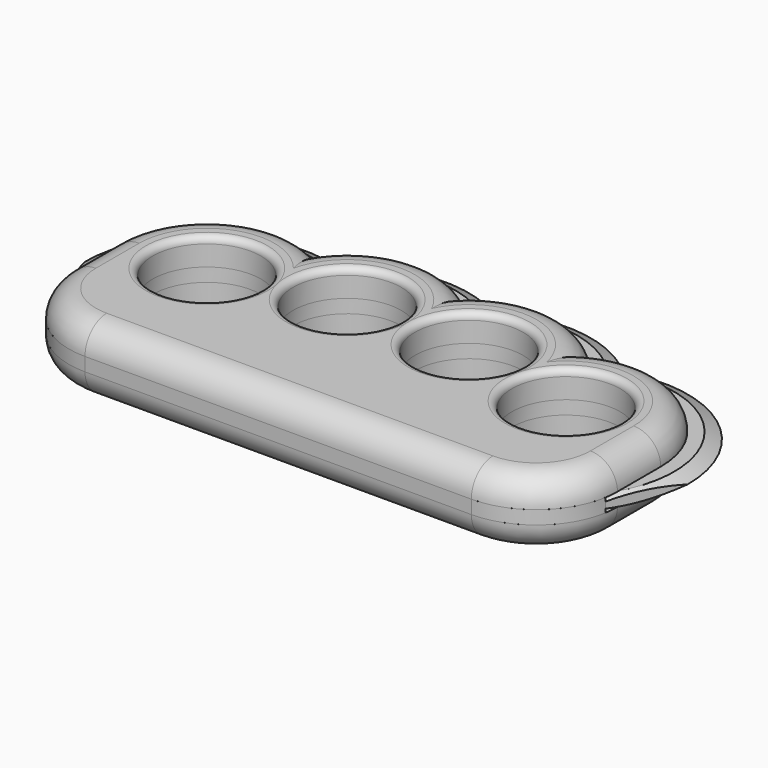
from build123d import *

# Parameters (mm, degrees)
F1_START = 1.5875
F0_R     = 12.7
F1_DEPTH = 6.35
F2_START = -1.5875
F2_DEPTH = 6.35
F3_R     = 12.7
F4_DEPTH = 3.175
F5_SIZE2 = 3.175
F5_SIZE  = 1.5875
F6_SIZE2 = 1.58749
F6_SIZE  = 3.17499
F7_DEPTH = 3.175
F8_R     = 6.34999
F8_2_R   = 6.34999
F9_R     = 1.58749
F9_2_R   = 1.58749


# Not quite as in the source:
# - a fillet or chamfer is up to 0.001 mm smaller than in the source, because OpenCascade refuses the exact size


with BuildPart() as f1:
    # F0 (on Top) → F1 (new body)
    with BuildSketch(Plane.XY.offset(F1_START)):
        with BuildLine():
            ThreePointArc((32.0008761662, 51.5233725194), (16.7725271795, 60.185634809), (0, 55.1240409054))
            ThreePointArc((0, 55.1240409054), (-16.7725271795, 60.185634809), (-32.0008761662, 51.5233725194))
            ThreePointArc((-32.0008761662, 51.5233725194), (-53.7331431906, 50.7166907676), (-64.37301193, 31.75))
            Line((-64.37301193, 31.75), (-64.37301193, 19.05))
            ThreePointArc((-64.37301193, 19.05), (-58.7933961116, 5.5796158184), (-45.32301193, 0))
            Line((-45.32301193, 0), (0, 0))
            Line((0, 0), (45.32301193, 0))
            ThreePointArc((45.32301193, 0), (58.7933961116, 5.5796158184), (64.37301193, 19.05))
            Line((64.37301193, 19.05), (64.37301193, 31.75))
            ThreePointArc((64.37301193, 31.75), (53.7331431906, 50.7166907676), (32.0008761662, 51.5233725194))
        make_face()
        with Locations((-42.14801193, 31.75)):
            Circle(F0_R, mode=Mode.SUBTRACT)
        with Locations((-14.2875, 38.1)):
            Circle(F0_R, mode=Mode.SUBTRACT)
        with Locations((14.2875, 38.1)):
            Circle(F0_R, mode=Mode.SUBTRACT)
        with Locations((42.14801193, 31.75)):
            Circle(F0_R, mode=Mode.SUBTRACT)
    extrude(amount=F1_DEPTH)

    # F8 (radius 6.35 in the source; OpenCascade refuses exactly that, so slightly less here)
    f8_edges = [f1.edges().sort_by_distance(p)[0] for p in [
        (-58.793396, 5.579616, 7.9375),
        (-64.373012, 25.4, 7.9375),
        (-53.733143, 50.716691, 7.9375),
        (-16.772527, 60.185635, 7.9375),
        (16.772527, 60.185635, 7.9375),
        (53.733143, 50.716691, 7.9375),
        (58.793396, 5.579616, 7.9375),
        (64.373012, 25.4, 7.9375),
        (0, 0, 7.9375),
    ]]
    fillet(f8_edges, radius=F8_R)

    # F9#2 (radius 1.5875 in the source; OpenCascade refuses exactly that, so slightly less here)
    f9_2_edges = [f1.edges().sort_by_distance(p)[0] for p in [
        (29.448012, 31.75, 7.9375),
        (1.5875, 38.1, 7.9375),
        (-26.9875, 38.1, 7.9375),
        (-54.848012, 31.75, 7.9375),
    ]]
    fillet(f9_2_edges, radius=F9_2_R)


with BuildPart() as f2:
    # F0 (on Top) → F2 (new body)
    with BuildSketch(Plane.XY.offset(F2_START)):
        with BuildLine():
            ThreePointArc((32.0008761662, 51.5233725194), (16.7725271795, 60.185634809), (0, 55.1240409054))
            ThreePointArc((0, 55.1240409054), (-16.7725271795, 60.185634809), (-32.0008761662, 51.5233725194))
            ThreePointArc((-32.0008761662, 51.5233725194), (-53.7331431906, 50.7166907676), (-64.37301193, 31.75))
            Line((-64.37301193, 31.75), (-64.37301193, 19.05))
            ThreePointArc((-64.37301193, 19.05), (-58.7933961116, 5.5796158184), (-45.32301193, 0))
            Line((-45.32301193, 0), (0, 0))
            Line((0, 0), (45.32301193, 0))
            ThreePointArc((45.32301193, 0), (58.7933961116, 5.5796158184), (64.37301193, 19.05))
            Line((64.37301193, 19.05), (64.37301193, 31.75))
            ThreePointArc((64.37301193, 31.75), (53.7331431906, 50.7166907676), (32.0008761662, 51.5233725194))
        make_face()
        with Locations((-42.14801193, 31.75)):
            Circle(F0_R, mode=Mode.SUBTRACT)
        with Locations((-14.2875, 38.1)):
            Circle(F0_R, mode=Mode.SUBTRACT)
        with Locations((14.2875, 38.1)):
            Circle(F0_R, mode=Mode.SUBTRACT)
        with Locations((42.14801193, 31.75)):
            Circle(F0_R, mode=Mode.SUBTRACT)
    extrude(amount=-F2_DEPTH)

    # F8#2 (radius 6.35 in the source; OpenCascade refuses exactly that, so slightly less here)
    f8_2_edges = [f2.edges().sort_by_distance(p)[0] for p in [
        (0, 0, -7.9375),
        (-64.373012, 25.4, -7.9375),
        (-16.772527, 60.185635, -7.9375),
        (-53.733143, 50.716691, -7.9375),
        (-58.793396, 5.579616, -7.9375),
        (16.772527, 60.185635, -7.9375),
        (53.733143, 50.716691, -7.9375),
        (64.373012, 25.4, -7.9375),
        (58.793396, 5.579616, -7.9375),
    ]]
    fillet(f8_2_edges, radius=F8_2_R)

    # F9 (radius 1.5875 in the source; OpenCascade refuses exactly that, so slightly less here)
    f9_edges = [f2.edges().sort_by_distance(p)[0] for p in [
        (-54.848012, 31.75, -7.9375),
        (-26.9875, 38.1, -7.9375),
        (1.5875, 38.1, -7.9375),
        (29.448012, 31.75, -7.9375),
    ]]
    fillet(f9_edges, radius=F9_R)


with BuildPart() as f4:
    # F3 (on face) → F4 (new body)
    with BuildSketch(Plane.XY.offset(-1.5875)):
        with BuildLine():
            Line((-70.72301193, 31.75), (-64.1065652413, 15.875))
            Line((-64.1065652413, 15.875), (64.1065652413, 15.875))
            Line((64.1065652413, 15.875), (70.72301193, 31.75))
            ThreePointArc((70.72301193, 31.75), (59.1129014499, 54.7439807031), (33.717017279, 59.0529110938))
            ThreePointArc((33.717017279, 59.0529110938), (17.4825349451, 66.495816183), (0, 62.8466759131))
            ThreePointArc((0, 62.8466759131), (-17.4825349451, 66.495816183), (-33.717017279, 59.0529110938))
            ThreePointArc((-33.717017279, 59.0529110938), (-59.1129014499, 54.7439807031), (-70.72301193, 31.75))
        make_face()
        with Locations((-42.14801193, 31.75)):
            Circle(F3_R, mode=Mode.SUBTRACT)
        with Locations((-14.2875, 38.1)):
            Circle(F3_R, mode=Mode.SUBTRACT)
        with Locations((14.2875, 38.1)):
            Circle(F3_R, mode=Mode.SUBTRACT)
        with Locations((42.14801193, 31.75)):
            Circle(F3_R, mode=Mode.SUBTRACT)
    extrude(amount=F4_DEPTH)

    # F5
    f5_edges = [f4.edges().sort_by_distance(p)[0] for p in [
        (-17.482535, 66.495816, -1.5875),
        (-59.112901, 54.743981, -1.5875),
        (17.482535, 66.495816, -1.5875),
        (59.112901, 54.743981, -1.5875),
    ]]
    chamfer(f5_edges, length=F5_SIZE, length2=F5_SIZE2)

    # F6 (size 3.175 and 1.5875 in the source; OpenCascade refuses exactly that, so slightly less here)
    f6_edges = [f4.edges().sort_by_distance(p)[0] for p in [
        (-59.112901, 54.743981, 1.5875),
        (-17.482535, 66.495816, 1.5875),
        (17.482535, 66.495816, 1.5875),
        (59.112901, 54.743981, 1.5875),
    ]]
    f6_side = f4.faces().sort_by_distance((0, 40.532073, 1.5875))[0]
    chamfer(f6_edges, length=F6_SIZE, length2=F6_SIZE2, reference=f6_side)


with BuildPart() as f7:
    # F3 (on face) → F7 (new body)
    with BuildSketch(Plane.XY.offset(-1.5875)):
        with BuildLine():
            Line((64.1065652413, 15.875), (-64.1065652413, 15.875))
            ThreePointArc((-64.1065652413, 15.875), (-57.6197340542, 4.5003221685), (-45.32301193, 0))
            Line((-45.32301193, 0), (45.32301193, 0))
            ThreePointArc((45.32301193, 0), (57.6197340542, 4.5003221685), (64.1065652413, 15.875))
        make_face()
    extrude(amount=F7_DEPTH)


solid = Compound([f1.part, f2.part, f4.part, f7.part])
